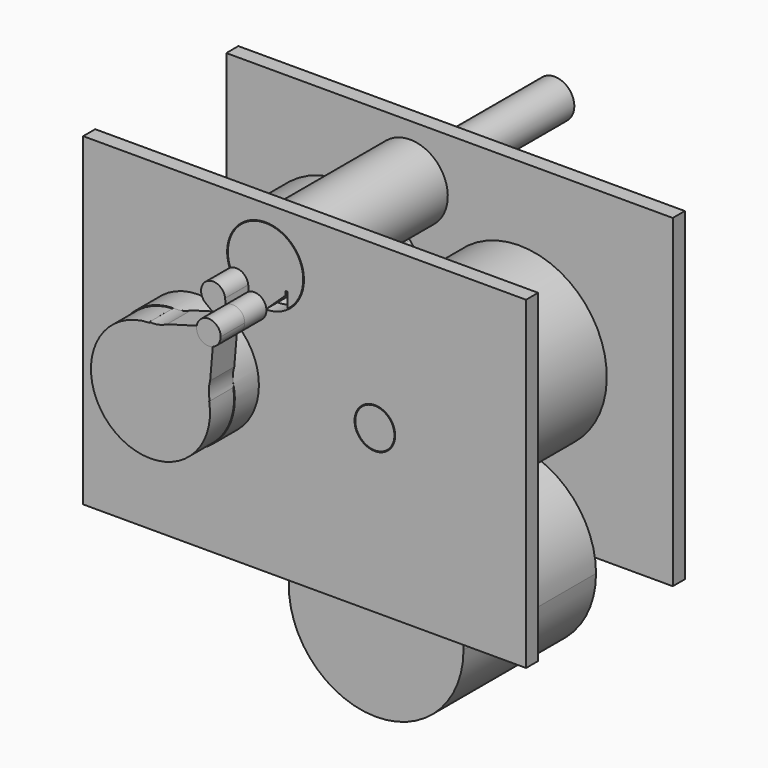
from build123d import *
from build123d import SkipClean  # not in build123d's __all__

# Parameters (mm, degrees)
F1_DEPTH  = 55
F2_DEPTH  = 55
F3_DEPTH  = 5
F4_W      = 147.0356285572
F4_H      = 107.6404266059
F4_R      = 12.75
F5_DEPTH  = 5
F6_R      = 6.5
F7_DEPTH  = 60
F6_R_2    = 6.37
F8_R      = 6.75
F8_R_2    = 6.5
F9_DEPTH  = 5
F10_W     = 148.2294239104
F10_H     = 107.6404303312
F10_R     = 29
F10_R_2   = 6.75
F11_DEPTH = 5
F12_R     = 20
F13_DEPTH = 10
F15_DEPTH = 9.6
F16_R     = 1.4667338037
F16_R_2   = 1.575645526
F17_DEPTH = 1
F19_DEPTH = 10
F20_R     = 4
F21_DEPTH = 19


# Not quite as in the source:
# - a feature names something its author has since deleted; it is built from what else it names


with BuildPart() as f1:
    # F0 (on Front) → F1 (new body)
    with BuildSketch(Plane.XZ):
        with BuildLine():
            ThreePointArc((-41.1536252148, 23.2401222417), (-42.0160454202, 23.8595733703), (-42.9005648719, 24.4470371146))
            ThreePointArc((-42.9005648719, 24.4470371146), (-83.9301358502, -13.9394472861), (-29.5, 0))
            ThreePointArc((-29.5, 0), (-30.3890739875, 7.1257167163), (-33.0017819808, 13.8145169241))
            ThreePointArc((-33.0017819808, 13.8145169241), (-34.5495422962, 16.3516230319), (-36.348838503, 18.7169988068))
            ThreePointArc((-36.348838503, 18.7169988068), (-38.6221604672, 21.1156694307), (-41.1536252148, 23.2401222417))
        make_face()
    extrude(amount=-F1_DEPTH)

    # F6 (on face) → F7, piece 2 (join, symmetric)
    with BuildSketch(Plane(origin=(0, 55, 0), x_dir=(-1, 0, 0), z_dir=(0, 1, 0))):
        with Locations((58.5, 0)):
            Circle(F6_R_2)
    extrude(amount=F7_DEPTH, both=True)

    # F12 (on face) → F13 (join)
    with BuildSketch(Plane.XZ.offset(5)):
        with Locations((-58.5, 0)):
            Circle(F12_R)
    extrude(amount=F13_DEPTH)

    # F16 (on face) → F17 (cut)
    with BuildSketch(Plane(origin=(0, 55, 0), x_dir=(-1, 0, 0), z_dir=(0, 1, 0))):
        with Locations((32.9697545245, 13.7552377646)):
            Circle(F16_R)
        with Locations((37.7860717411, 20.2961369745)):
            Circle(F16_R_2)
    extrude(amount=-F17_DEPTH, mode=Mode.SUBTRACT)

    # F18 (on face) → F19 (join)
    with BuildSketch(Plane.XZ.offset(15)):
        with BuildLine():
            Line((-58.8650048174, 19.9966690097), (-58.8650048174, 19.7679851447))
            ThreePointArc((-58.8650048174, 19.7679851447), (-71.0876028348, -15.2465969997), (-39.0204476237, 3.3843026488))
            Line((-39.0204476237, 3.3843026488), (-38.7958999198, 3.4275997474))
            ThreePointArc((-38.7958999198, 3.4275997474), (-39.158784575, 6.4252112319), (-38.6819540845, 9.4068202888))
            Line((-38.6819540845, 9.4068202888), (-37.8152522193, 19.6275492174))
            ThreePointArc((-37.8152522193, 19.6275492174), (-41.7427232808, 20.2970691325), (-43.1437283838, 24.0267434556))
            Line((-43.1437283838, 24.0267434556), (-53.0155028424, 21.2406097555))
            ThreePointArc((-53.0155028424, 21.2406097555), (-55.852904996, 20.207890576), (-58.8650048174, 19.9966690097))
        make_face()
        with BuildLine():
            ThreePointArc((-35.1960889101, 23.3816523105), (-38.8724825867, 27.3685406896), (-43.1437283838, 24.0267434556))
            ThreePointArc((-43.1437283838, 24.0267434556), (-41.7427232808, 20.2970691325), (-37.8152522193, 19.6275492174))
            ThreePointArc((-37.8152522193, 19.6275492174), (-35.915589957, 21.0929132213), (-35.1960889101, 23.3816523105))
        make_face()
    extrude(amount=F19_DEPTH)

    # F20 (on face) → F21 (join)
    with BuildSketch(Plane.XZ.offset(25)):
        with Locations((-39.1960889101, 23.3816523105)):
            Circle(F20_R)
    with SkipClean():  # cleaning this boolean's faces spoils the solid; the shape is the same uncleaned
        extrude(amount=-F21_DEPTH)


with BuildPart() as f1b:
    # F0 (on Front) → F1, piece 2 (new body)
    with BuildSketch(Plane.XZ):
        with BuildLine():
            ThreePointArc((-28.9684026443, 1.3533839956), (-28.9920995849, 0.676876398), (-29, 0))
            ThreePointArc((-29, 0), (28.6408007806, -4.5502231426), (-27.5721013347, 8.9877265196))
            ThreePointArc((-27.5721013347, 8.9877265196), (-28.5267934404, 5.217476019), (-28.9684026443, 1.3533839956))
        make_face()
    extrude(amount=-F1_DEPTH)

    # F6 (on face) → F7 (join, symmetric)
    with BuildSketch(Plane(origin=(0, 55, 0), x_dir=(-1, 0, 0), z_dir=(0, 1, 0))):
        Circle(F6_R)
    extrude(amount=F7_DEPTH, both=True)


with BuildPart() as f1c:
    # F0 (on Front) → F1, piece 3 (new body)
    with BuildSketch(Plane.XZ):
        with BuildLine():
            ThreePointArc((-8.5874367907, -30.0348162964), (-6.6181195056, -33.6613095975), (-5.9369329363, -37.7314016223))
            ThreePointArc((-5.9369329363, -37.7314016223), (-14.8949027207, -49.7190628601), (-28.9295764486, -44.5251069533))
            ThreePointArc((-28.9295764486, -44.5251069533), (-10.8414991929, -86.6723671252), (25.4269504417, -58.5980080068))
            ThreePointArc((25.4269504417, -58.5980080068), (20.1416741432, -41.9063370372), (6.2123380445, -31.2988104094))
            ThreePointArc((6.2123380445, -31.2988104094), (-1.1052506579, -29.703199328), (-8.5874367907, -30.0348162964))
        make_face()
    extrude(amount=-F1_DEPTH)

    # F0 (on Front) → F2, piece 2 (join)
    with BuildSketch(Plane.XZ):
        with BuildLine():
            ThreePointArc((-28.9295764486, -44.5251069533), (-14.8949027207, -49.7190628601), (-5.9369329363, -37.7314016223))
            ThreePointArc((-5.9369329363, -37.7314016223), (-6.6181195056, -33.6613095975), (-8.5874367907, -30.0348162964))
            ThreePointArc((-8.5874367907, -30.0348162964), (-20.398335202, -34.9778944802), (-28.9295764486, -44.5251069533))
        make_face()
    extrude(amount=-F2_DEPTH)


with BuildPart() as f2:
    # F0 (on Front) → F2 (new body)
    with BuildSketch(Plane.XZ):
        with BuildLine():
            Line((-29.7499911844, 29.0422718972), (-29.7499911844, 30.4551975319))
            Line((-29.7499911844, 30.4551975319), (-29.0499911844, 30.4551975319))
            Line((-29.0499911844, 30.4551975319), (-29.0499911844, 28.7470832982))
            Line((-29.0499911844, 28.7470832982), (-29.0499911844, 25.4551975319))
            ThreePointArc((-29.0499911844, 25.4551975319), (-37.2019757379, 48.111576961), (-41.9707706725, 24.5102003937))
            ThreePointArc((-41.9707706725, 24.5102003937), (-39.0674891647, 23.4573161705), (-35.9946793142, 23.148369049))
            Line((-35.9946793142, 23.148369049), (-29.7499911844, 29.0422718972))
        make_face()
    extrude(amount=-F2_DEPTH)

    # F3 (add): a face of the model
    f3_faces = [f2.faces().sort_by_distance(p)[0] for p in [
        (-36.4766460991, 0, 36.0174252396),
    ]]
    extrude(f3_faces, amount=F3_DEPTH)

    # F6 (on face) → F7, piece 3 (join, symmetric)
    with BuildSketch(Plane(origin=(0, 55, 0), x_dir=(-1, 0, 0), z_dir=(0, 1, 0))):
        with Locations((36.2901888608, 35.6448755251)):
            Circle(F6_R)
    extrude(amount=F7_DEPTH, both=True)

    # F14 (on face) → F15 (join)
    with BuildSketch(Plane.XZ.offset(5)):
        with BuildLine():
            Line((-41.5423475849, 23.2477869574), (-42.039366708, 28.1814121262))
            ThreePointArc((-42.039366708, 28.1814121262), (-42.0411706118, 28.1997414844), (-42.0430588933, 28.2180623422))
            ThreePointArc((-42.0430588933, 28.2180623422), (-47.0802039077, 31.6560257646), (-49.6552624965, 26.1277805045))
            ThreePointArc((-49.6552624965, 26.1277805045), (-49.1521463113, 25.3096121307), (-48.4684965177, 24.6349653021))
            Line((-48.4684965177, 24.6349653021), (-44.6557707015, 21.6855334745))
            ThreePointArc((-44.6557707015, 21.6855334745), (-42.5611405388, 21.3946394228), (-41.5423475849, 23.2477869574))
        make_face()
    extrude(amount=F15_DEPTH)


with BuildPart() as f5:
    # F4 (on face) → F5 (new body)
    with BuildSketch(Plane.XZ):
        with Locations((-23.3261063695, 0.0221710652)):
            Rectangle(F4_W, F4_H)
        with Locations((-36.2901888608, 35.6448755251)):
            Circle(F4_R, mode=Mode.SUBTRACT)
    extrude(amount=F5_DEPTH)

    # F8 (on face) → F9 (cut)
    with BuildSketch(Plane.XZ.offset(5)):
        Circle(F8_R)
        with Locations((-58.5, 0)):
            Circle(F8_R)
        with Locations((-36.2901888608, 35.6448755251)):
            Circle(F8_R_2)
    extrude(amount=-F9_DEPTH, mode=Mode.SUBTRACT)


with BuildPart() as f11:
    # F10 (on face) → F11 (new body)
    with BuildSketch(Plane(origin=(0, 55, 0), x_dir=(-1, 0, 0), z_dir=(0, 1, 0))):
        with Locations((23.2089590281, -0.2336390316)):
            Rectangle(F10_W, F10_H)
        Circle(F10_R, mode=Mode.SUBTRACT)
        with Locations((58.5, 0)):
            Circle(F10_R_2, mode=Mode.SUBTRACT)
        with Locations((36.2901888608, 35.6448755251)):
            Circle(F10_R_2, mode=Mode.SUBTRACT)
        Circle(F10_R)
        Circle(F10_R_2, mode=Mode.SUBTRACT)
    extrude(amount=F11_DEPTH)


solid = Compound([f1.part, f1b.part, f1c.part, f2.part, f5.part, f11.part])
